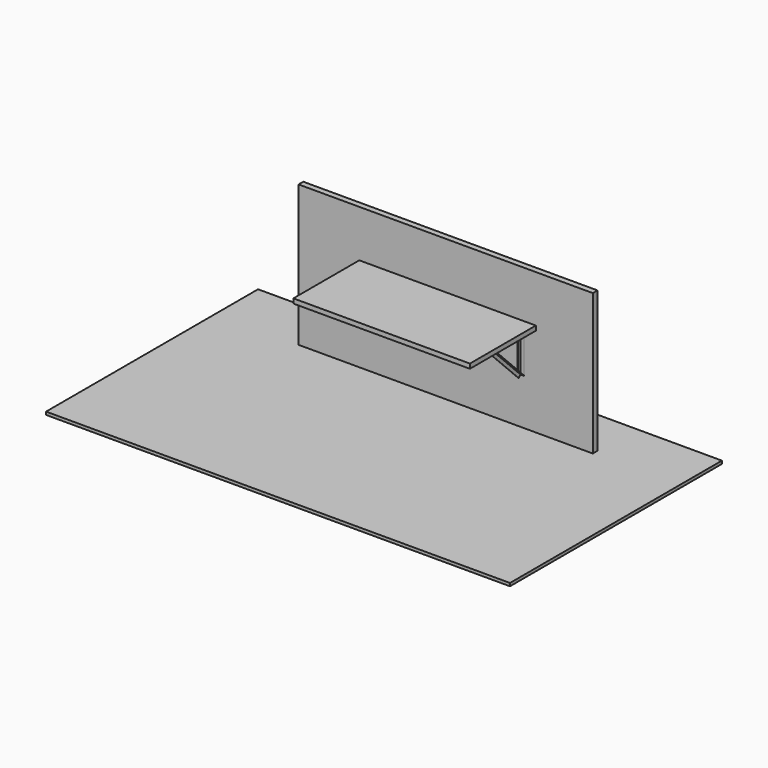
from build123d import *

# Parameters (mm, degrees)
F0_W      = 2500
F0_H      = 1200
F1_DEPTH  = 50
F2_W      = 3941.5423870087
F2_H      = 2251.1970996857
F3_DEPTH  = 25
F5_W      = 1500
F5_H      = 700
F6_DEPTH  = 39
F7_W      = 500
F7_H      = 45
F8_DEPTH  = 45
F10_DEPTH = 550
F12_DEPTH = 368
F15_REACH = 1880.5875140627


with BuildPart() as f1:
    # F0 (on Front) → F1 (new body)
    with BuildSketch(Plane.XZ):
        with Locations((1250, 600)):
            Rectangle(F0_W, F0_H)
    extrude(amount=-F1_DEPTH)


with BuildPart() as f3:
    # F2 (on Top) → F3 (new body)
    with BuildSketch(Plane.XY):
        with Locations((1261.9167566299, -669.9469089508)):
            Rectangle(F2_W, F2_H)
    extrude(amount=-F3_DEPTH)


with BuildPart() as f6:
    # F5 (on offset) → F6 (new body)
    with BuildSketch(Plane.XY.offset(800)):
        with Locations((1265.8117413521, -350)):
            Rectangle(F5_W, F5_H)
    extrude(amount=-F6_DEPTH)


with BuildPart() as f8:
    # F7 (on face) → F8 (new body)
    with BuildSketch(Plane.XZ):
        with Locations((1265.8117413521, 738.5)):
            Rectangle(F7_W, F7_H)
    extrude(amount=F8_DEPTH)


with BuildPart() as f10:
    # F9 (on face) → F10 (new body)
    with BuildSketch(Plane.XZ):
        Polygon((645.8117413521, 761), (615.8117413521, 761), (615.8117413521, 758), (642.8117413521, 758), (642.8117413521, 731), (645.8117413521, 731), align=None)
    extrude(amount=F10_DEPTH)


with BuildPart() as f10b:
    # F9 (on face) → F10, piece 2 (new body)
    with BuildSketch(Plane.XZ):
        Polygon((1915.8117413521, 758), (1915.8117413521, 761), (1885.8117413521, 761), (1885.8117413521, 731), (1888.8117413521, 731), (1888.8117413521, 758), align=None)
    extrude(amount=F10_DEPTH)


with BuildPart() as f12:
    # F11 (on face) → F12 (new body)
    with BuildSketch(Plane(origin=(0, 0, 761), x_dir=(1, 0, 0), z_dir=(0, 0, -1))):
        Polygon((615.6302545255, 2.9945053902), (615.8117413521, 0), (645.8117413521, 0), (645.8117413521, 30), (642.8117413521, 30), (642.8117413521, 2.9945053902), align=None)
    extrude(amount=F12_DEPTH)


with BuildPart() as f12b:
    # F11 (on face) → F12, piece 2 (new body)
    with BuildSketch(Plane(origin=(0, 0, 761), x_dir=(1, 0, 0), z_dir=(0, 0, -1))):
        Polygon((1888.8117413521, 30), (1885.8117413521, 30), (1885.8117413521, 0), (1915.8117413521, 0), (1915.8117413521, 3), (1888.8117413521, 3), align=None)
    extrude(amount=F12_DEPTH)


with BuildPart() as f15:
    f15_end = Plane(origin=(629.3117413521, -275, 758), x_dir=(-1, 0, 0), z_dir=(0, 0, -1))
    # F14 (on face) → F15 (new body, up to a plane its end follows)
    with BuildSketch(Plane(origin=(0, -197.9972526951, 197.9972526951), x_dir=(1, 0, 0), z_dir=(0, -0.7071067812, 0.7071067812))):
        Polygon((642.6302545255, 248.7755299386), (645.6302545255, 248.7755299386), (645.6302545255, 278.7755299386), (615.6302545255, 278.7755299386), (615.6302545255, 275.7755299386), (642.6302545255, 275.7755299386), align=None)
    f15_long = extrude(amount=F15_REACH, mode=Mode.PRIVATE)
    add(split(f15_long, bisect_by=f15_end, keep=Keep.TOP, mode=Mode.PRIVATE))


with BuildPart() as f15b:
    f15_2_end = Plane(origin=(629.3117413521, -275, 758), x_dir=(-1, 0, 0), z_dir=(0, 0, -1))
    # F14 (on face) → F15, piece 2 (new body, up to a plane its end follows)
    with BuildSketch(Plane(origin=(0, -197.9972526951, 197.9972526951), x_dir=(1, 0, 0), z_dir=(0, -0.7071067812, 0.7071067812))):
        Polygon((1915.8117413521, 275.7716446628), (1915.8117413521, 278.7716446628), (1885.8117413521, 278.7716446628), (1885.8117413521, 248.7716446628), (1888.8117413521, 248.7716446628), (1888.8117413521, 275.7716446628), align=None)
    f15_2_long = extrude(amount=F15_REACH, mode=Mode.PRIVATE)
    add(split(f15_2_long, bisect_by=f15_2_end, keep=Keep.TOP, mode=Mode.PRIVATE))


solid = Compound([f1.part, f3.part, f6.part, f8.part, f10.part, f10b.part, f12.part, f12b.part, f15.part, f15b.part])
